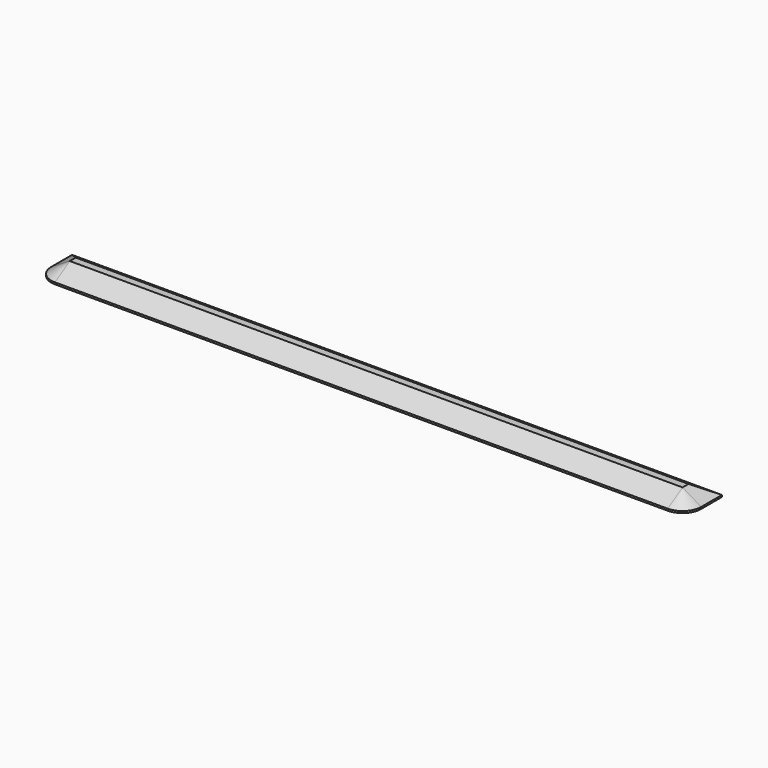
from build123d import *

# Parameters (mm, degrees)
F1_DEPTH = 3.5
F2_SIZE2 = 2.99999
F2_SIZE  = 4.99999


# Not quite as in the source:
# - a fillet or chamfer is up to 0.001 mm smaller than in the source, because OpenCascade refuses the exact size


with BuildPart() as f1:
    # F0 (on Top) → F1 (new body)
    with BuildSketch(Plane.XY):
        with BuildLine():
            Line((-82.5, -6), (82.5, -6))
            ThreePointArc((82.5, -6), (86.0355339059, -4.5355339059), (87.5, -1))
            Line((87.5, -1), (87.5, 6))
            Line((87.5, 6), (-87.5, 6))
            Line((-87.5, 6), (-87.5, -1))
            ThreePointArc((-87.5, -1), (-86.0355339059, -4.5355339059), (-82.5, -6))
        make_face()
    extrude(amount=F1_DEPTH)

    # F2 (size 5 and 3 in the source; OpenCascade refuses exactly that, so slightly less here)
    f2_edges = [f1.edges().sort_by_distance(p)[0] for p in [
        (0, 6, 3.5),
        (87.5, 2.5, 3.5),
    ]]
    f2_side = f1.faces().sort_by_distance((0, 0.025079, 3.5))[0]
    chamfer(f2_edges, length=F2_SIZE, length2=F2_SIZE2, reference=f2_side)


solid = f1.part
